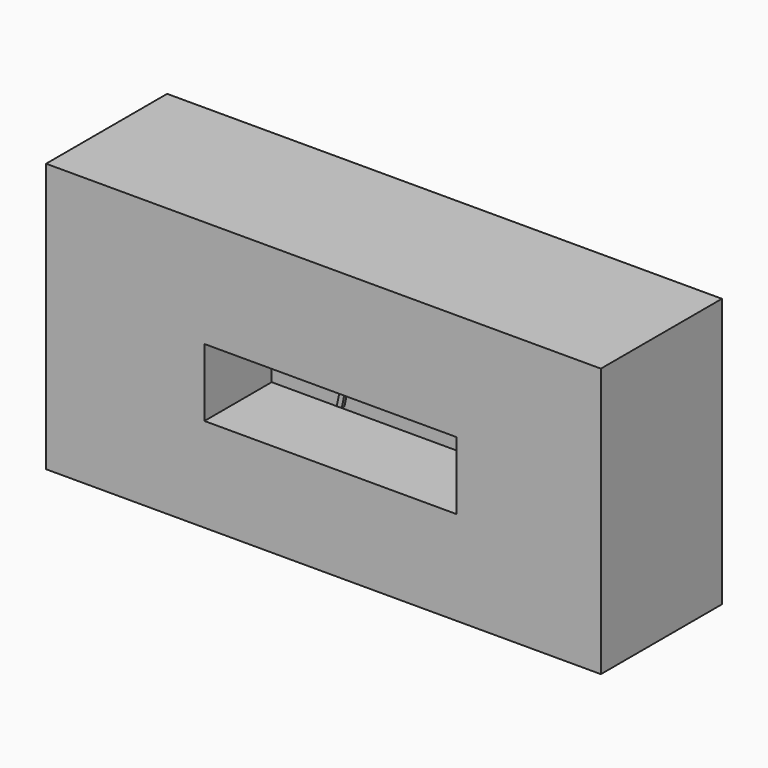
from build123d import *

# Parameters (mm, degrees)
F0_W         = 209.55
F0_H         = 101.6
F1_DEPTH     = 57.15
F3_W         = 95.1392911375
F3_H         = 25.6079277024
F4_DEPTH     = 57.15
F5_TEXT_SIZE = 23.8296983298
F6_DEPTH     = 1.27


# Not quite as in the source:
# - Text() gives the source's letters only with a copy of the font that has no kerning and outlines rounded to 1/6400 em; it was checked with that copy


with BuildPart() as f1:
    # F0 (on Front) → F1 (new body)
    with BuildSketch(Plane.XZ):
        with Locations((7.6785814017, 2.0680310541)):
            Rectangle(F0_W, F0_H)
    extrude(amount=F1_DEPTH)

    # F3 (on offset) → F4 (cut)
    with BuildSketch(Plane.XZ.offset(25.4)):
        with Locations((10.2859865874, -0.4311040975)):
            Rectangle(F3_W, F3_H)
    extrude(amount=F4_DEPTH, mode=Mode.SUBTRACT)

    # F5 (on offset) → F6 (join)
    with BuildSketch(Plane.XZ.offset(25.4)):
        with Locations((-36.9374742731, -6.6814832389)):
            Text('Supreme', F5_TEXT_SIZE, font='Open Sans', font_style=FontStyle.ITALIC, text_align=(TextAlign.LEFT, TextAlign.BOTTOM))
    extrude(amount=F6_DEPTH)


solid = f1.part
